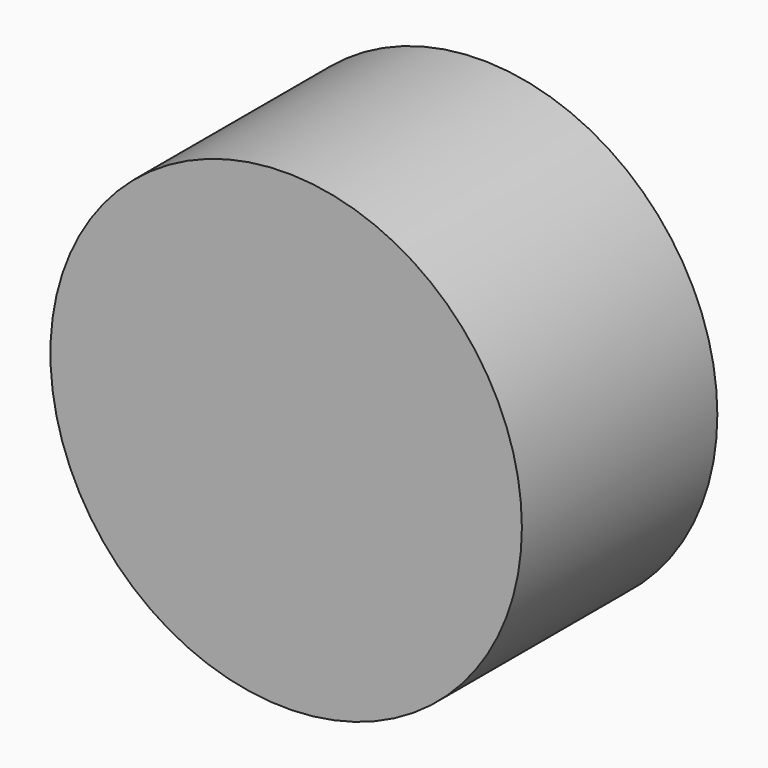
from build123d import *

# Parameters (mm, degrees)
F0_R     = 128.8146505864
F1_DEPTH = 25.4
F3_R     = 49.0141215923
F4_DEPTH = 50.8


# Not quite as in the source:
# - the program builds the solid bodies; features that only make, move or delete a surface that nothing else refers to are left out


with BuildPart() as f1:
    # F0 (on Front) → F1 (new body)
    with BuildSketch(Plane.XZ):
        with Locations((10.3380498641, 23.791786507)):
            Circle(F0_R)
        with BuildLine():
            ThreePointArc((48.5750728322, 28.0582736708), (55.5999914747, 14.8036448721), (58.026257129, 0))
            ThreePointArc((58.026257129, 0), (42.1859059552, -34.9036707218), (5.4861297438, -45.9630279004))
            ThreePointArc((5.4861297438, -45.9630279004), (-66.466433543, -36.001514495), (-48.743487455, 34.4420820545))
            ThreePointArc((-48.743487455, 34.4420820545), (0.9542816207, 81.3053730097), (48.7808239875, 32.5338840485))
            ThreePointArc((48.7808239875, 32.5338840485), (48.7293590503, 30.2937154281), (48.5750728322, 28.0582736708))
        make_face(mode=Mode.SUBTRACT)
    extrude(amount=F1_DEPTH)


with BuildPart() as f4:
    # F3 (on Front) → F4 (new body)
    with BuildSketch(Plane.XZ):
        Circle(F3_R)
    extrude(amount=F4_DEPTH)


solid = f4.part
